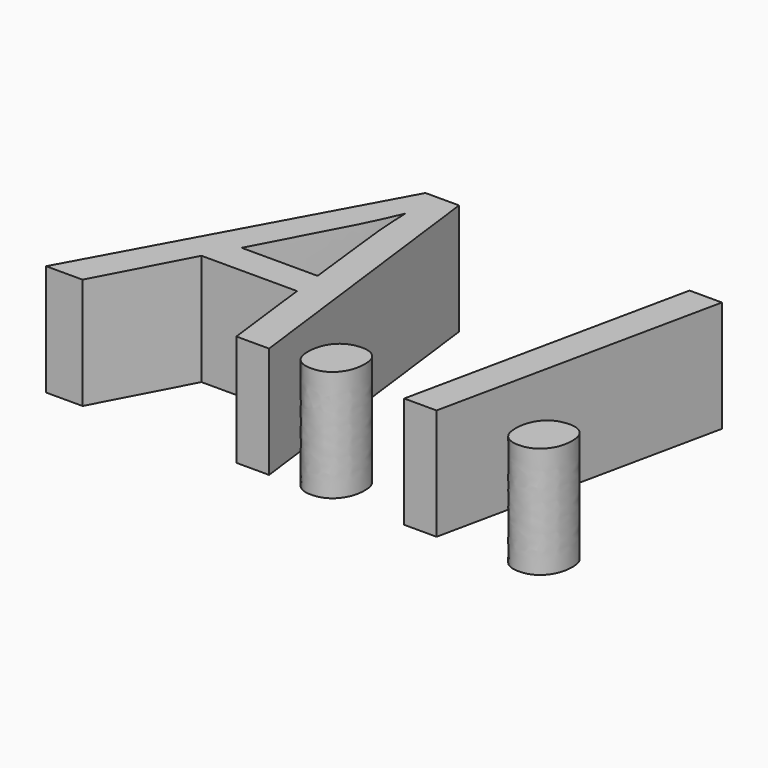
from build123d import *

# Parameters (mm, degrees)
F0_TEXT_SIZE = 18.0260019584
F1_DEPTH     = 5.08


# Not quite as in the source:
# - Text() gives the source's letters only with a copy of the font that has no kerning and outlines rounded to 1/6400 em; it was checked with that copy


with BuildPart() as f1:
    # F0 (on Top) → F1 (new body)
    with BuildSketch(Plane.XY):
        with Locations((-24.2477891968, 0)):
            Text('A.I.', F0_TEXT_SIZE, font='Open Sans', font_style=FontStyle.ITALIC, text_align=(TextAlign.LEFT, TextAlign.BOTTOM))
    extrude(amount=F1_DEPTH)


solid = f1.part
